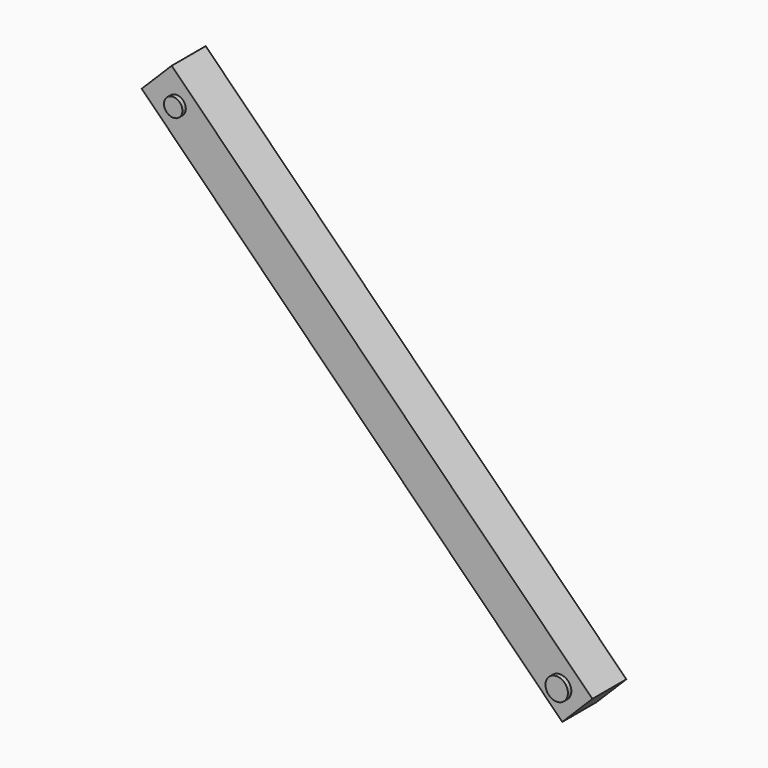
from build123d import *

# Parameters (mm, degrees)
F1_DEPTH = 10
F2_R     = 2.6409813422
F2_R_2   = 2.1665688489
F3_DEPTH = 1


# Not quite as in the source:
# - a feature names something its author has since deleted; it is built from what else it names


with BuildPart() as f1:
    # F0 (on Front) → F1 (new body)
    with BuildSketch(Plane.XZ):
        Polygon((-49.4838858729, 98.9949493661), (-56.5549536848, 91.9238815543), (42.4399956814, -7.0710678119), (49.5110634932, 0), align=None)
    extrude(amount=F1_DEPTH)

    # F2 (on face) → F3 (join)
    with BuildSketch(Plane.XZ.offset(10)):
        with Locations((41.9252365828, 0)):
            Circle(F2_R)
        with Locations((-48.3359694481, 91.1623910069)):
            Circle(F2_R_2)
    extrude(amount=F3_DEPTH)


solid = f1.part
